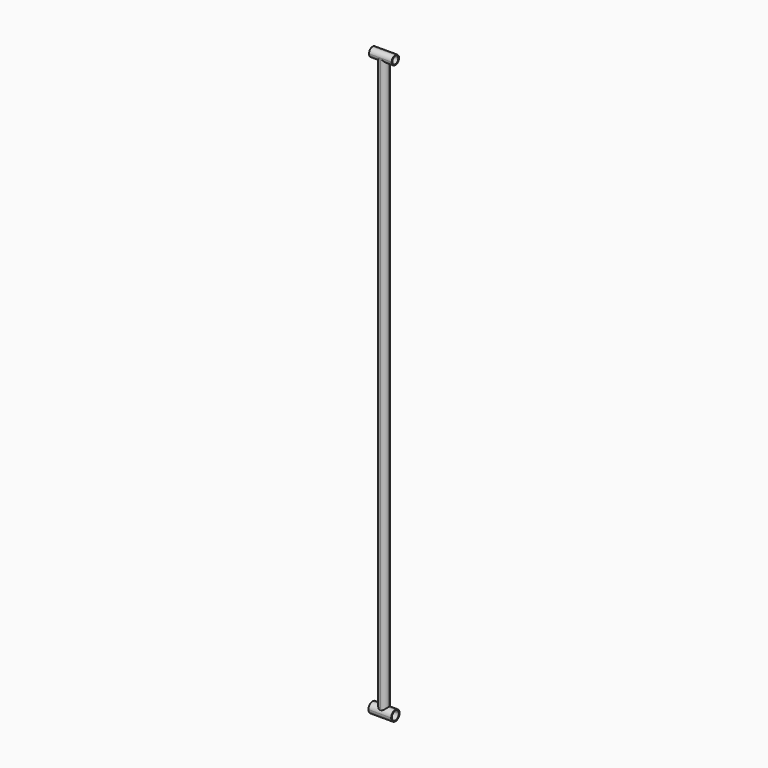
from build123d import *

# Parameters (mm, degrees)
F0_W         = 20
F0_H         = 1249.13
F0_W_2       = 50
F0_H_2       = 16
F0_H_3       = 2
F1_DEPTH     = 10
F0_H_4       = 19
F2_DEPTH     = 11.5
F3_DEPTH     = 9.5
F4_DEPTH     = 8
F5_R         = 7.99999
F6_R         = 9.49999
F7_T1_DEPTH  = 107.4995000022
F7_T6_DEPTH  = 107.4995000022
F7_T12_DEPTH = 107.4995000022
F7_T18_DEPTH = 107.4995000022
F7_T25_DEPTH = 107.4995000022
F7_T31_DEPTH = 107.4995000022
F7_T37_DEPTH = 107.4995000022
F7_T43_DEPTH = 107.4995000022
F7_T49_DEPTH = 107.4995000022
F7_T56_DEPTH = 107.4995000022
F7_T62_DEPTH = 107.4995000022
F8_R         = 9.99999


# Not quite as in the source:
# - a fillet or chamfer that OpenCascade refuses, or shapes differently, is made with other operations: its cross-section is extruded or revolved along the edge and cut away or added
# - a fillet or chamfer is up to 0.001 mm smaller than in the source, because OpenCascade refuses the exact size


with BuildPart() as f1:
    # F0 (on Front) → F1 (new body, symmetric)
    with BuildSketch(Plane.XZ):
        with Locations((25, 647.565)):
            Rectangle(F0_W, F0_H)
        Polygon((0, 1272.13), (15, 1272.13), (35, 1272.13), (50, 1272.13), (50, 1274.13), (0, 1274.13), align=None)
        with Locations((25, 1282.13)):
            Rectangle(F0_W_2, F0_H_2)
        with Locations((25, 1291.13)):
            Rectangle(F0_W_2, F0_H_3)
    extrude(amount=F1_DEPTH, both=True)

    # F0 (on Front) → F2 (join, symmetric)
    with BuildSketch(Plane.XZ):
        Polygon((0, 23), (0, 21), (50, 21), (50, 23), (35, 23), (15, 23), align=None)
        with Locations((25, 11.5)):
            Rectangle(F0_W_2, F0_H_4)
        with Locations((25, 1)):
            Rectangle(F0_W_2, F0_H_3)
    extrude(amount=F2_DEPTH, both=True)

    # F0 (on Front) → F3 (cut, symmetric)
    with BuildSketch(Plane.XZ):
        with Locations((25, 11.5)):
            Rectangle(F0_W_2, F0_H_4)
    extrude(amount=F3_DEPTH, both=True, mode=Mode.SUBTRACT)

    # F0 (on Front) → F4 (cut, symmetric)
    with BuildSketch(Plane.XZ):
        with Locations((25, 1282.13)):
            Rectangle(F0_W_2, F0_H_2)
    extrude(amount=F4_DEPTH, both=True, mode=Mode.SUBTRACT)

    # F5 (radius 8 in the source; OpenCascade refuses exactly that, so slightly less here)
    f5_edges = [f1.edges().sort_by_distance(p)[0] for p in [
        (25, -8, 1290.13),
        (25, -8, 1274.13),
        (25, 8, 1274.13),
        (25, 8, 1290.13),
    ]]
    fillet(f5_edges, radius=F5_R)

    # F6 (radius 9.5 in the source; OpenCascade refuses exactly that, so slightly less here)
    f6_edges = [f1.edges().sort_by_distance(p)[0] for p in [
        (25, 9.5, 2),
        (25, -9.5, 2),
        (25, -9.5, 21),
        (25, 9.5, 21),
    ]]
    fillet(f6_edges, radius=F6_R)

    # F7: fillet of radius 11.5 on 4 edges, made by hand

    # F7_s2 → F7_t1 (cut)
    with BuildSketch(Plane.YZ.offset(-28.7497500011)):
        with BuildLine():
            ThreePointArc((-0.0001, -0.0001), (-8.1318279836, 3.3681720164), (-11.5001, 11.4999))
            Line((-11.5001, 11.4999), (-11.7301, 11.4999))
            ThreePointArc((-11.7301, 11.4999), (-11.73, 5.74995), (-11.73, 0))
            Line((-11.73, 0), (-11.5, -0.23))
            ThreePointArc((-11.5, -0.23), (-5.75005, -0.23), (-0.0001, -0.2301))
            Line((-0.0001, -0.2301), (-0.0001, -0.0001))
        make_face()
        with BuildLine():
            ThreePointArc((0.0001, -0.0001), (8.1318279836, 3.3681720164), (11.5001, 11.4999))
            Line((11.5001, 11.4999), (11.7301, 11.4999))
            ThreePointArc((11.7301, 11.4999), (11.73, 5.74995), (11.73, 0))
            Line((11.73, 0), (11.5, -0.23))
            ThreePointArc((11.5, -0.23), (5.75005, -0.23), (0.0001, -0.2301))
            Line((0.0001, -0.2301), (0.0001, -0.0001))
        make_face()
    extrude(amount=F7_T1_DEPTH, mode=Mode.SUBTRACT)


with BuildPart() as f7_tool4:
    # F7_s5 → F7_t6 (new body)
    with BuildSketch(Plane.YZ.offset(78.7497500011)):
        with BuildLine():
            ThreePointArc((-11.5001, 11.5001), (-8.1318279836, 19.6318279836), (-0.0001, 23.0001))
            Line((-0.0001, 23.0001), (-0.0001, 23.2301))
            ThreePointArc((-0.0001, 23.2301), (-5.75005, 23.23), (-11.5, 23.23))
            Line((-11.5, 23.23), (-11.73, 23))
            ThreePointArc((-11.73, 23), (-11.73, 17.25005), (-11.7301, 11.5001))
            Line((-11.7301, 11.5001), (-11.5001, 11.5001))
        make_face()
    extrude(amount=-F7_T6_DEPTH)

    split(bisect_by=Plane.XZ.offset(10), keep=Keep.TOP)

    split(bisect_by=Plane.YZ.offset(35), keep=Keep.TOP)


with BuildPart() as f1_1:
    add(f1.part)

    # F7_t3: cut F7_tool4
    add(f7_tool4.part, mode=Mode.SUBTRACT)


with BuildPart() as f7_tool10:
    # F7_s11 → F7_t12 (new body)
    with BuildSketch(Plane.YZ.offset(78.7497500011)):
        with BuildLine():
            ThreePointArc((-11.5001, 11.5001), (-8.1318279836, 19.6318279836), (-0.0001, 23.0001))
            Line((-0.0001, 23.0001), (-0.0001, 23.2301))
            ThreePointArc((-0.0001, 23.2301), (-5.75005, 23.23), (-11.5, 23.23))
            Line((-11.5, 23.23), (-11.73, 23))
            ThreePointArc((-11.73, 23), (-11.73, 17.25005), (-11.7301, 11.5001))
            Line((-11.7301, 11.5001), (-11.5001, 11.5001))
        make_face()
    extrude(amount=-F7_T12_DEPTH)

    split(bisect_by=Plane.XZ.offset(10), keep=Keep.BOTTOM)

    split(bisect_by=Plane.YZ.offset(35), keep=Keep.TOP)


with BuildPart() as f1_2:
    add(f1_1.part)

    # F7_t9: cut F7_tool10
    add(f7_tool10.part, mode=Mode.SUBTRACT)


with BuildPart() as f7_tool16:
    # F7_s17 → F7_t18 (new body)
    with BuildSketch(Plane.YZ.offset(78.7497500011)):
        with BuildLine():
            ThreePointArc((-11.5001, 11.5001), (-8.1318279836, 19.6318279836), (-0.0001, 23.0001))
            Line((-0.0001, 23.0001), (-0.0001, 23.2301))
            ThreePointArc((-0.0001, 23.2301), (-5.75005, 23.23), (-11.5, 23.23))
            Line((-11.5, 23.23), (-11.73, 23))
            ThreePointArc((-11.73, 23), (-11.73, 17.25005), (-11.7301, 11.5001))
            Line((-11.7301, 11.5001), (-11.5001, 11.5001))
        make_face()
    extrude(amount=-F7_T18_DEPTH)

    split(bisect_by=Plane.YZ.offset(15), keep=Keep.TOP)

    split(bisect_by=Plane.XZ.offset(10), keep=Keep.TOP)

    split(bisect_by=Plane.YZ.offset(35), keep=Keep.BOTTOM)


with BuildPart() as f1_3:
    add(f1_2.part)

    # F7_t15: cut F7_tool16
    add(f7_tool16.part, mode=Mode.SUBTRACT)


with BuildPart() as f7_tool23:
    # F7_s24 → F7_t25 (new body)
    with BuildSketch(Plane.YZ.offset(78.7497500011)):
        with BuildLine():
            ThreePointArc((-11.5001, 11.5001), (-8.1318279836, 19.6318279836), (-0.0001, 23.0001))
            Line((-0.0001, 23.0001), (-0.0001, 23.2301))
            ThreePointArc((-0.0001, 23.2301), (-5.75005, 23.23), (-11.5, 23.23))
            Line((-11.5, 23.23), (-11.73, 23))
            ThreePointArc((-11.73, 23), (-11.73, 17.25005), (-11.7301, 11.5001))
            Line((-11.7301, 11.5001), (-11.5001, 11.5001))
        make_face()
    extrude(amount=-F7_T25_DEPTH)

    split(bisect_by=Plane.YZ.offset(15), keep=Keep.BOTTOM)

    split(bisect_by=Plane.XZ.offset(10), keep=Keep.TOP)


with BuildPart() as f1_4:
    add(f1_3.part)

    # F7_t22: cut F7_tool23
    add(f7_tool23.part, mode=Mode.SUBTRACT)


with BuildPart() as f7_tool29:
    # F7_s30 → F7_t31 (new body)
    with BuildSketch(Plane.YZ.offset(78.7497500011)):
        with BuildLine():
            ThreePointArc((-11.5001, 11.5001), (-8.1318279836, 19.6318279836), (-0.0001, 23.0001))
            Line((-0.0001, 23.0001), (-0.0001, 23.2301))
            ThreePointArc((-0.0001, 23.2301), (-5.75005, 23.23), (-11.5, 23.23))
            Line((-11.5, 23.23), (-11.73, 23))
            ThreePointArc((-11.73, 23), (-11.73, 17.25005), (-11.7301, 11.5001))
            Line((-11.7301, 11.5001), (-11.5001, 11.5001))
        make_face()
    extrude(amount=-F7_T31_DEPTH)

    split(bisect_by=Plane.YZ.offset(15), keep=Keep.BOTTOM)

    split(bisect_by=Plane.XZ.offset(10), keep=Keep.BOTTOM)


with BuildPart() as f1_5:
    add(f1_4.part)

    # F7_t28: cut F7_tool29
    add(f7_tool29.part, mode=Mode.SUBTRACT)


with BuildPart() as f7_tool35:
    # F7_s36 → F7_t37 (new body)
    with BuildSketch(Plane.YZ.offset(78.7497500011)):
        with BuildLine():
            ThreePointArc((11.5001, 11.5001), (8.1318279836, 19.6318279836), (0.0001, 23.0001))
            Line((0.0001, 23.0001), (0.0001, 23.2301))
            ThreePointArc((0.0001, 23.2301), (5.75005, 23.23), (11.5, 23.23))
            Line((11.5, 23.23), (11.73, 23))
            ThreePointArc((11.73, 23), (11.73, 17.25005), (11.7301, 11.5001))
            Line((11.7301, 11.5001), (11.5001, 11.5001))
        make_face()
    extrude(amount=-F7_T37_DEPTH)

    split(bisect_by=Plane.YZ.offset(35), keep=Keep.TOP)

    split(bisect_by=Plane.XZ.offset(-10), keep=Keep.BOTTOM)


with BuildPart() as f1_6:
    add(f1_5.part)

    # F7_t34: cut F7_tool35
    add(f7_tool35.part, mode=Mode.SUBTRACT)


with BuildPart() as f7_tool41:
    # F7_s42 → F7_t43 (new body)
    with BuildSketch(Plane.YZ.offset(78.7497500011)):
        with BuildLine():
            ThreePointArc((11.5001, 11.5001), (8.1318279836, 19.6318279836), (0.0001, 23.0001))
            Line((0.0001, 23.0001), (0.0001, 23.2301))
            ThreePointArc((0.0001, 23.2301), (5.75005, 23.23), (11.5, 23.23))
            Line((11.5, 23.23), (11.73, 23))
            ThreePointArc((11.73, 23), (11.73, 17.25005), (11.7301, 11.5001))
            Line((11.7301, 11.5001), (11.5001, 11.5001))
        make_face()
    extrude(amount=-F7_T43_DEPTH)

    split(bisect_by=Plane.YZ.offset(35), keep=Keep.TOP)

    split(bisect_by=Plane.XZ.offset(-10), keep=Keep.TOP)


with BuildPart() as f1_7:
    add(f1_6.part)

    # F7_t40: cut F7_tool41
    add(f7_tool41.part, mode=Mode.SUBTRACT)


with BuildPart() as f7_tool47:
    # F7_s48 → F7_t49 (new body)
    with BuildSketch(Plane.YZ.offset(78.7497500011)):
        with BuildLine():
            ThreePointArc((11.5001, 11.5001), (8.1318279836, 19.6318279836), (0.0001, 23.0001))
            Line((0.0001, 23.0001), (0.0001, 23.2301))
            ThreePointArc((0.0001, 23.2301), (5.75005, 23.23), (11.5, 23.23))
            Line((11.5, 23.23), (11.73, 23))
            ThreePointArc((11.73, 23), (11.73, 17.25005), (11.7301, 11.5001))
            Line((11.7301, 11.5001), (11.5001, 11.5001))
        make_face()
    extrude(amount=-F7_T49_DEPTH)

    split(bisect_by=Plane.YZ.offset(15), keep=Keep.TOP)

    split(bisect_by=Plane.YZ.offset(35), keep=Keep.BOTTOM)

    split(bisect_by=Plane.XZ.offset(-10), keep=Keep.BOTTOM)


with BuildPart() as f1_8:
    add(f1_7.part)

    # F7_t46: cut F7_tool47
    add(f7_tool47.part, mode=Mode.SUBTRACT)


with BuildPart() as f7_tool54:
    # F7_s55 → F7_t56 (new body)
    with BuildSketch(Plane.YZ.offset(78.7497500011)):
        with BuildLine():
            ThreePointArc((11.5001, 11.5001), (8.1318279836, 19.6318279836), (0.0001, 23.0001))
            Line((0.0001, 23.0001), (0.0001, 23.2301))
            ThreePointArc((0.0001, 23.2301), (5.75005, 23.23), (11.5, 23.23))
            Line((11.5, 23.23), (11.73, 23))
            ThreePointArc((11.73, 23), (11.73, 17.25005), (11.7301, 11.5001))
            Line((11.7301, 11.5001), (11.5001, 11.5001))
        make_face()
    extrude(amount=-F7_T56_DEPTH)

    split(bisect_by=Plane.YZ.offset(15), keep=Keep.BOTTOM)

    split(bisect_by=Plane.XZ.offset(-10), keep=Keep.BOTTOM)


with BuildPart() as f1_9:
    add(f1_8.part)

    # F7_t53: cut F7_tool54
    add(f7_tool54.part, mode=Mode.SUBTRACT)


with BuildPart() as f7_tool60:
    # F7_s61 → F7_t62 (new body)
    with BuildSketch(Plane.YZ.offset(78.7497500011)):
        with BuildLine():
            ThreePointArc((11.5001, 11.5001), (8.1318279836, 19.6318279836), (0.0001, 23.0001))
            Line((0.0001, 23.0001), (0.0001, 23.2301))
            ThreePointArc((0.0001, 23.2301), (5.75005, 23.23), (11.5, 23.23))
            Line((11.5, 23.23), (11.73, 23))
            ThreePointArc((11.73, 23), (11.73, 17.25005), (11.7301, 11.5001))
            Line((11.7301, 11.5001), (11.5001, 11.5001))
        make_face()
    extrude(amount=-F7_T62_DEPTH)

    split(bisect_by=Plane.YZ.offset(15), keep=Keep.BOTTOM)

    split(bisect_by=Plane.XZ.offset(-10), keep=Keep.TOP)


with BuildPart() as f1_10:
    add(f1_9.part)

    # F7_t59: cut F7_tool60
    add(f7_tool60.part, mode=Mode.SUBTRACT)

    # F8 (radius 10 in the source; OpenCascade refuses exactly that, so slightly less here)
    f8_edges = [f1_10.edges().sort_by_distance(p)[0] for p in [
        (7.5, -10, 1272.13),
        (25, -10, 1292.13),
        (42.5, -10, 1272.13),
        (35, -10, 644.654592),
        (15, -10, 644.654592),
        (35, 10, 644.654592),
        (42.5, 10, 1272.13),
        (25, 10, 1292.13),
        (15, 10, 644.654592),
        (7.5, 10, 1272.13),
    ]]
    fillet(f8_edges, radius=F8_R)


solid = f1_10.part
